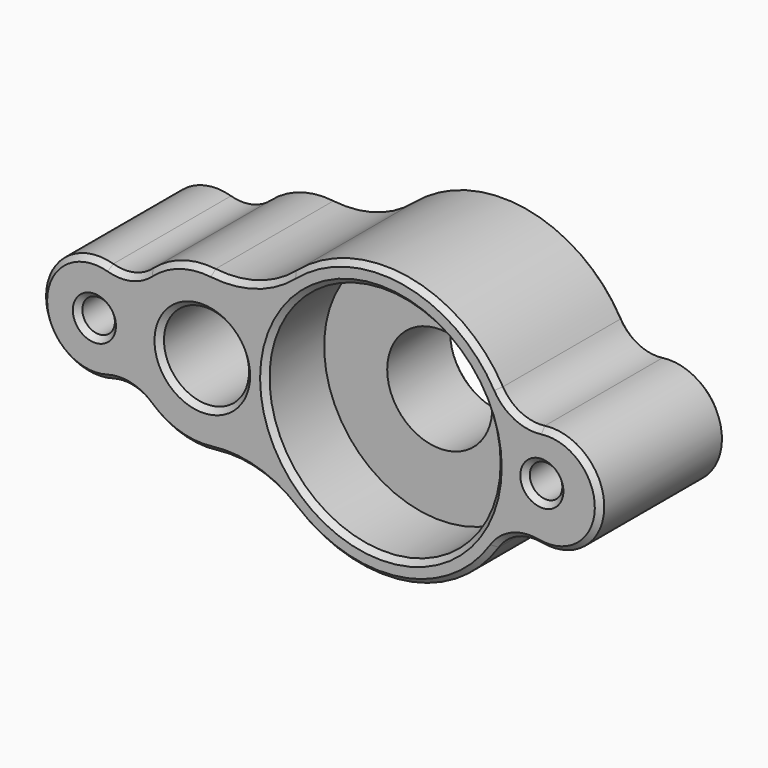
from build123d import *

# Parameters (mm, degrees)
F1_R     = 1.5499996566
F1_R_2   = 4.05
F1_R_3   = 11
F2_DEPTH = 15
F3_R     = 1.5499996566
F3_R_2   = 11
F3_R_3   = 4.05
F3_R_4   = 5
F4_DEPTH = 8
F5_SIZE  = 0.5


# Not quite as in the source:
# - a feature names something its author has since deleted; it is built from what else it names


with BuildPart() as f2:
    # F1 (on offset) → F2 (new body)
    with BuildSketch(Plane.XZ.offset(7.5)):
        with BuildLine():
            ThreePointArc((-16.1097446178, 5.6510393794), (-17.8915523622, 4.7319149036), (-19.8955278727, 4.792831184))
            ThreePointArc((-19.8955278727, 4.792831184), (-26.2950637706, 0.0064660896), (-19.9219776461, -4.815061031))
            ThreePointArc((-19.9219776461, -4.815061031), (-17.917697117, -4.7651791649), (-16.1409768963, -5.694099989))
            ThreePointArc((-16.1409768963, -5.694099989), (-13.3010298936, -7.316379445), (-10.0427278071, -7.6002053168))
            ThreePointArc((-10.0427278071, -7.6002053168), (-5.9542872002, -7.917007121), (-2.3367475524, -9.848099267))
            ThreePointArc((-2.3367475524, -9.848099267), (7.8678117277, -12.7279820224), (16.8033240158, -7.0197971151))
            ThreePointArc((16.8033240158, -7.0197971151), (18.58751675, -5.5306692402), (20.898442998, -5.2847720721))
            ThreePointArc((20.898442998, -5.2847720721), (26.8344703592, -0.5175206843), (21.1826859269, 4.5835026796))
            ThreePointArc((21.1826859269, 4.5835026796), (18.8897447965, 4.9620083109), (17.1942238361, 6.5513648516))
            ThreePointArc((17.1942238361, 6.5513648516), (8.1466571288, 12.85030216), (-2.4748372324, 9.8975183761))
            ThreePointArc((-2.4748372324, 9.8975183761), (-6.0650144321, 7.9160195357), (-10.1486242942, 7.5420670334))
            ThreePointArc((-10.1486242942, 7.5420670334), (-13.3318829255, 7.2355232201), (-16.1097446178, 5.6510393794))
        make_face()
        with Locations((-21.2950828407, -0.0072984656)):
            Circle(F1_R, mode=Mode.SUBTRACT)
        with Locations((-11.0252965242, -0.0355703814)):
            Circle(F1_R_2, mode=Mode.SUBTRACT)
        with Locations((21.2950848365, -0.0073001884)):
            Circle(F1_R, mode=Mode.SUBTRACT)
        with Locations((5.9747034758, 0.0833180019)):
            Circle(F1_R_3, mode=Mode.SUBTRACT)
    extrude(amount=-F2_DEPTH)

    # F3 (on face) → F4 (join)
    with BuildSketch(Plane(origin=(0, 7.5, 0), x_dir=(-1, 0, 0), z_dir=(0, 1, 0))):
        with BuildLine():
            ThreePointArc((10.1486242942, 7.5420670334), (6.0650144321, 7.9160195357), (2.4748372324, 9.8975183761))
            ThreePointArc((2.4748372324, 9.8975183761), (-8.1466571288, 12.85030216), (-17.1942238361, 6.5513648516))
            ThreePointArc((-17.1942238361, 6.5513648516), (-18.8897447965, 4.9620083109), (-21.1826859269, 4.5835026796))
            ThreePointArc((-21.1826859269, 4.5835026796), (-26.8344703592, -0.5175206843), (-20.898442998, -5.2847720721))
            ThreePointArc((-20.898442998, -5.2847720721), (-18.58751675, -5.5306692402), (-16.8033240158, -7.0197971151))
            ThreePointArc((-16.8033240158, -7.0197971151), (-7.8678117277, -12.7279820224), (2.3367475524, -9.848099267))
            ThreePointArc((2.3367475524, -9.848099267), (5.9542872002, -7.917007121), (10.0427278071, -7.6002053168))
            ThreePointArc((10.0427278071, -7.6002053168), (13.3010298936, -7.316379445), (16.1409768963, -5.694099989))
            ThreePointArc((16.1409768963, -5.694099989), (17.917697117, -4.7651791649), (19.9219776461, -4.815061031))
            ThreePointArc((19.9219776461, -4.815061031), (26.2950637706, 0.0064660896), (19.8955278727, 4.792831184))
            ThreePointArc((19.8955278727, 4.792831184), (17.8915523622, 4.7319149036), (16.1097446178, 5.6510393794))
            ThreePointArc((16.1097446178, 5.6510393794), (13.3318829255, 7.2355232201), (10.1486242942, 7.5420670334))
        make_face()
        with Locations((-21.2950848365, -0.0073001884)):
            Circle(F3_R, mode=Mode.SUBTRACT)
        with Locations((-5.9747034758, 0.0833180019)):
            Circle(F3_R_2, mode=Mode.SUBTRACT)
        with Locations((11.0252965242, -0.0355703814)):
            Circle(F3_R_3, mode=Mode.SUBTRACT)
        with Locations((21.2950828407, -0.0072984656)):
            Circle(F3_R, mode=Mode.SUBTRACT)
        with Locations((-5.9747034758, 0.0833180019)):
            Circle(F3_R_2)
        with Locations((-5.9747034758, 0.0833180019)):
            Circle(F3_R_4, mode=Mode.SUBTRACT)
    extrude(amount=-F4_DEPTH)

    # F5
    f5_edges = [f2.edges().sort_by_distance(p)[0] for p in [
        (-6.065014, -7.5, 7.91602),
        (8.146657, -7.5, 12.850302),
        (18.889745, -7.5, 4.962008),
        (26.83447, -7.5, -0.517521),
        (18.587517, -7.5, -5.530669),
        (7.867812, -7.5, -12.727982),
        (-5.954287, -7.5, -7.917007),
        (-13.30103, -7.5, -7.316379),
        (-17.917697, -7.5, -4.765179),
        (-26.295064, -7.5, 0.006466),
        (-17.891552, -7.5, 4.731915),
        (-13.331883, -7.5, 7.235523),
        (-5.025297, -7.5, 0.083318),
        (-22.845082, -7.5, -0.007298),
        (19.745085, -7.5, -0.0073),
        (8.146657, 7.5, 12.850302),
        (-22.845082, 7.5, -0.007298),
        (10.974703, 7.5, 0.083318),
        (19.745085, 7.5, -0.0073),
        (-15.075297, -7.5, -0.03557),
        (-6.065014, 7.5, 7.91602),
        (-13.331883, 7.5, 7.235523),
        (-17.891552, 7.5, 4.731915),
        (-26.295064, 7.5, 0.006466),
        (-17.917697, 7.5, -4.765179),
        (-13.30103, 7.5, -7.316379),
        (-5.954287, 7.5, -7.917007),
        (7.867812, 7.5, -12.727982),
        (18.587517, 7.5, -5.530669),
        (26.83447, 7.5, -0.517521),
        (18.889745, 7.5, 4.962008),
    ]]
    chamfer(f5_edges, length=F5_SIZE)


solid = f2.part
